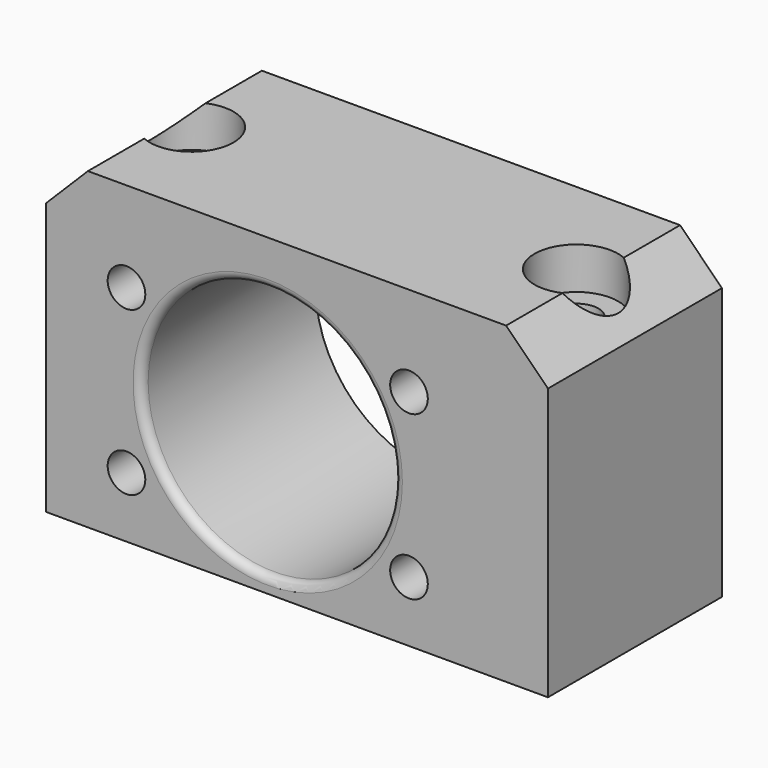
from build123d import *

# Parameters (mm, degrees)
F0_W           = 60
F0_H           = 37.5
F0_R           = 2.25
F0_R_2         = 15.1
F1_DEPTH       = 26
F3_D           = 5.3
F3_CBORE_D     = 10
F3_CBORE_DEPTH = 5
F4_T1_DEPTH    = 51.7168298797
F5_R           = 1


# Not quite as in the source:
# - a fillet or chamfer that OpenCascade refuses, or shapes differently, is made with other operations: its cross-section is extruded or revolved along the edge and cut away or added


with BuildPart() as f1:
    # F0 (on Front) → F1 (new body)
    with BuildSketch(Plane.XZ):
        with Locations((0, 1.25)):
            Rectangle(F0_W, F0_H)
        with Locations((-20.3874953738, -10.25)):
            Circle(F0_R, mode=Mode.SUBTRACT)
        with Locations((-3.5, -0.5)):
            Circle(F0_R_2, mode=Mode.SUBTRACT)
        with Locations((13.3874953738, -10.25)):
            Circle(F0_R, mode=Mode.SUBTRACT)
        with Locations((-20.3874953738, 9.25)):
            Circle(F0_R, mode=Mode.SUBTRACT)
        with Locations((13.3874953738, 9.25)):
            Circle(F0_R, mode=Mode.SUBTRACT)
    extrude(amount=-F1_DEPTH)

    # F3 (through all)
    with Locations(Plane.XY.offset(20)):
        with Locations((-23, 13), (23, 13)):
            CounterBoreHole(F3_D / 2, F3_CBORE_D / 2, F3_CBORE_DEPTH)

    # F4: chamfer of 5 on 2 edges, made by hand

    # F4_s2 → F4_t1 (cut)
    with BuildSketch(Plane.XZ.offset(-38.8584149398)):
        Polygon((-30, 15), (-25, 20), (-30, 20), align=None)
        Polygon((30, 15), (25, 20), (30, 20), align=None)
    extrude(amount=F4_T1_DEPTH, mode=Mode.SUBTRACT)

    # F5
    f5_edges = [f1.edges().sort_by_distance(p)[0] for p in [
        (-18.6, 0, -0.5),
    ]]
    fillet(f5_edges, radius=F5_R)


solid = f1.part
